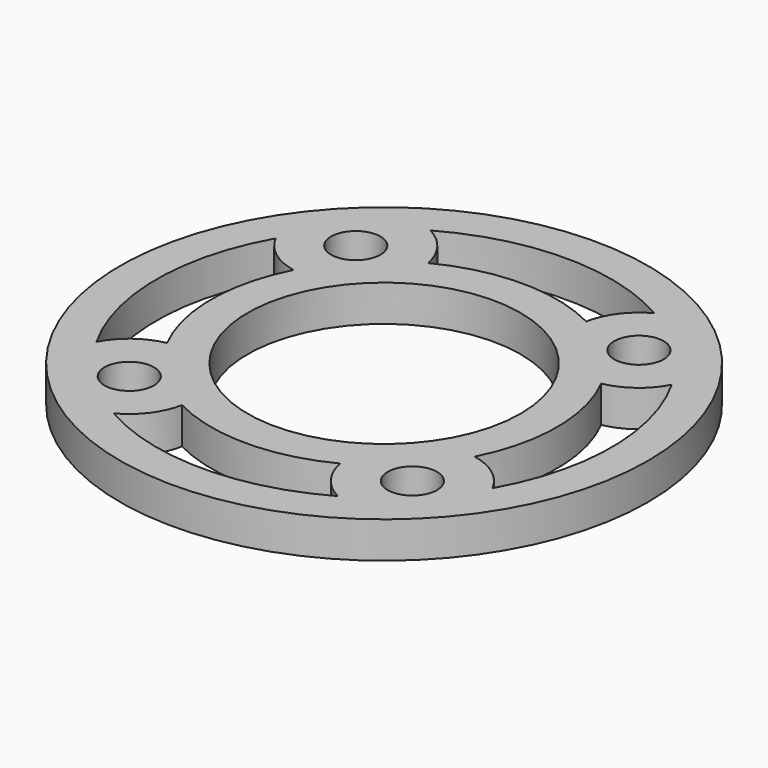
from build123d import *

# Parameters (mm, degrees)
F0_R            = 23.01875
F0_R_2          = 2.15265
F0_R_3          = 11.90625
F1_DEPTH        = 3.175
F3_DEPTH        = 3.175
F3_COPIES_COUNT = 4


# Not quite as in the source:
# - a pattern or mirror of a feature is missing from the dataset's text; its kind, count and spacing are read off the source's solid


with BuildPart() as f1:
    # F0 (on Top) → F1 (new body)
    with BuildSketch(Plane.XY):
        Circle(F0_R)
        with Locations((-12.3478521665, -12.3478521665)):
            Circle(F0_R_2, mode=Mode.SUBTRACT)
        with Locations((12.3478521665, -12.3478521665)):
            Circle(F0_R_2, mode=Mode.SUBTRACT)
        with Locations((-12.3478521665, 12.3478521665)):
            Circle(F0_R_2, mode=Mode.SUBTRACT)
        Circle(F0_R_3, mode=Mode.SUBTRACT)
        with Locations((12.3478521665, 12.3478521665)):
            Circle(F0_R_2, mode=Mode.SUBTRACT)
    extrude(amount=F1_DEPTH)

    # F2 (on face) → F3 (cut, through all)
    with BuildSketch(Plane.XY.offset(3.175)):
        with BuildLine():
            ThreePointArc((-9.7719120136, 17.2709047146), (-7.8938999882, 15.6696324205), (-6.8946489019, 13.4129757356))
            ThreePointArc((-6.8946489019, 13.4129757356), (0, 15.08125), (6.8946489019, 13.4129757356))
            ThreePointArc((6.8946489019, 13.4129757356), (7.8938999882, 15.6696324205), (9.7719120136, 17.2709047146))
            ThreePointArc((9.7719120136, 17.2709047146), (0, 19.84375), (-9.7719120136, 17.2709047146))
        make_face()
    f3 = extrude(amount=-F3_DEPTH, mode=Mode.SUBTRACT)

    # F3_copies: F3 ×4 about axis
    f3_copies_axis = Axis((0, 0, 0), (0, 0, 1))
    for i in range(1, F3_COPIES_COUNT):
        add(f3.rotate(f3_copies_axis, i * 360 / F3_COPIES_COUNT), mode=Mode.SUBTRACT)


solid = f1.part
